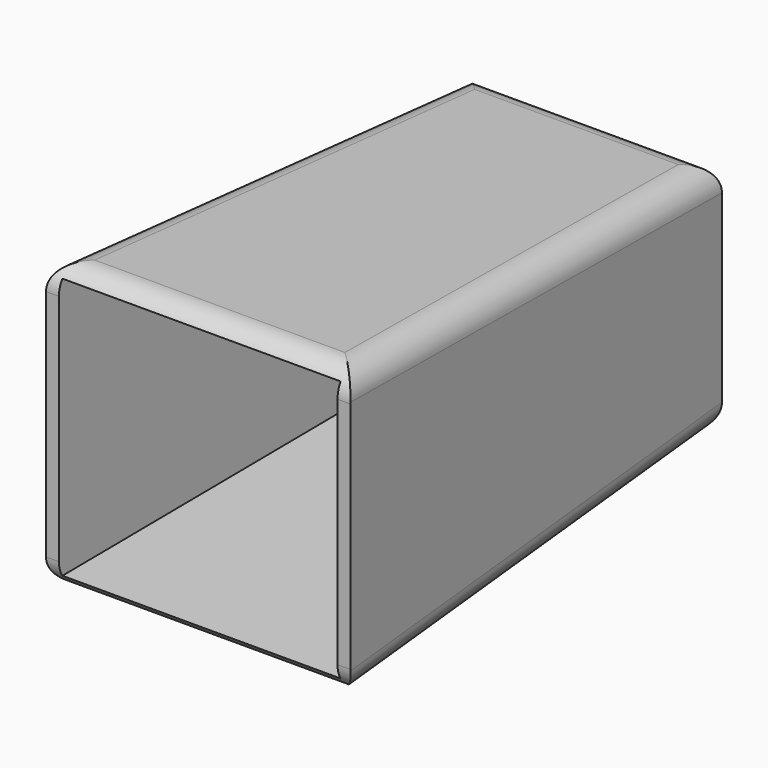
from build123d import *

# Parameters (mm, degrees)
F0_W        = 50
F0_H        = 46.7033070608
F1_DEPTH    = 98.552
F1_TAPER    = -3
F2_T        = -2.54
F3_T1_DEPTH = 74.1036999946
F3_T3_DEPTH = 124.1528328785
F3_T5_DEPTH = 87.0957981099
F3_T7_DEPTH = 124.1528328785
F4_T1_DEPTH = 74.1036999946
F4_T3_DEPTH = 124.1528328785
F4_T5_DEPTH = 87.0957981099
F4_T7_DEPTH = 124.1528328785


# Not quite as in the source:
# - a fillet or chamfer that OpenCascade refuses, or shapes differently, is made with other operations: its cross-section is extruded or revolved along the edge and cut away or added


with BuildPart() as f1:
    # F0 (on Front) → F1 (new body)
    with BuildSketch(Plane.XZ):
        Rectangle(F0_W, F0_H)
    extrude(amount=F1_DEPTH, taper=F1_TAPER)

    # F2
    f2_openings = [f1.faces().sort_by_distance(p)[0] for p in [
        (0, -98.552, 0),
    ]]
    offset(amount=F2_T, openings=f2_openings)

    # F3: fillet of radius 5.08 on 4 edges, made by hand

    # F3_s2 → F3_t1 (cut)
    with BuildSketch(Plane.YZ.offset(-37.0518499973)):
        with BuildLine():
            ThreePointArc((-4.8141333423, 23.6039515681), (-1.3950981953, 22.027754776), (0, 18.5309135315))
            Line((0, 18.5309135315), (0, 23.3516535304))
            Line((0, 23.3516535304), (-4.8141333423, 23.6039515681))
        make_face()
    extrude(amount=F3_T1_DEPTH, mode=Mode.SUBTRACT)

    # F3_s4 → F3_t3 (cut)
    with BuildSketch(Plane(origin=(0.5298667006, 10.1104589396, -0.5298667006), x_dir=(0.9986295348, -0.0523359562, 0), z_dir=(-0.0522644277, -0.9972646886, 0.0522644277))):
        with BuildLine():
            ThreePointArc((-24.9657383689, 18.1852510398), (-23.4827569315, 21.7724306367), (-19.8996527546, 23.2652319837))
            Line((-19.8996527546, 23.2652319837), (-24.9657383689, 23.2513556581))
            Line((-24.9657383689, 23.2513556581), (-24.9657383689, 18.1852510398))
        make_face()
    extrude(amount=F3_T3_DEPTH, mode=Mode.SUBTRACT)

    # F3_s6 → F3_t5 (cut)
    with BuildSketch(Plane.YZ.offset(-43.547899055)):
        with BuildLine():
            ThreePointArc((-93.2061333423, 28.2363799944), (-96.9688412445, 26.8482437626), (-98.552, 23.1633419579))
            Line((-98.552, 23.1633419579), (-98.552, 28.5165449943))
            Line((-98.552, 28.5165449943), (-93.2061333423, 28.2363799944))
        make_face()
    extrude(amount=F3_T5_DEPTH, mode=Mode.SUBTRACT)

    # F3_s8 → F3_t7 (cut)
    with BuildSketch(Plane(origin=(-0.5298667006, 10.1104589396, -0.5298667006), x_dir=(0.9986295348, 0.0523359562, 0), z_dir=(0.0522644277, -0.9972646886, 0.0522644277))):
        with BuildLine():
            ThreePointArc((24.9657383689, 18.1852510398), (23.4827569315, 21.7724306367), (19.8996527546, 23.2652319837))
            Line((19.8996527546, 23.2652319837), (24.9657383689, 23.2513556581))
            Line((24.9657383689, 23.2513556581), (24.9657383689, 18.1852510398))
        make_face()
    extrude(amount=F3_T7_DEPTH, mode=Mode.SUBTRACT)

    # F4: fillet of radius 5.08 on 4 edges, made by hand

    # F4_s2 → F4_t1 (cut)
    with BuildSketch(Plane.YZ.offset(-37.0518499973)):
        with BuildLine():
            ThreePointArc((-4.8141333423, -23.6039515681), (-1.3950981953, -22.027754776), (0, -18.5309135315))
            Line((0, -18.5309135315), (0, -23.3516535304))
            Line((0, -23.3516535304), (-4.8141333423, -23.6039515681))
        make_face()
    extrude(amount=F4_T1_DEPTH, mode=Mode.SUBTRACT)

    # F4_s4 → F4_t3 (cut)
    with BuildSketch(Plane(origin=(-0.5298667006, 10.1104589396, 0.5298667006), x_dir=(0.9986295348, 0.0523359562, 0), z_dir=(0.0522644277, -0.9972646886, -0.0522644277))):
        with BuildLine():
            ThreePointArc((19.8996527546, -23.2652319837), (23.4827569315, -21.7724306367), (24.9657383689, -18.1852510398))
            Line((24.9657383689, -18.1852510398), (24.9657383689, -23.2513556581))
            Line((24.9657383689, -23.2513556581), (19.8996527546, -23.2652319837))
        make_face()
    extrude(amount=F4_T3_DEPTH, mode=Mode.SUBTRACT)

    # F4_s6 → F4_t5 (cut)
    with BuildSketch(Plane.YZ.offset(-43.547899055)):
        with BuildLine():
            ThreePointArc((-98.552, -23.1633419579), (-96.9688412445, -26.8482437626), (-93.2061333423, -28.2363799944))
            Line((-93.2061333423, -28.2363799944), (-98.552, -28.5165449943))
            Line((-98.552, -28.5165449943), (-98.552, -23.1633419579))
        make_face()
    extrude(amount=F4_T5_DEPTH, mode=Mode.SUBTRACT)

    # F4_s8 → F4_t7 (cut)
    with BuildSketch(Plane(origin=(0.5298667006, 10.1104589396, 0.5298667006), x_dir=(0.9986295348, -0.0523359562, 0), z_dir=(-0.0522644277, -0.9972646886, -0.0522644277))):
        with BuildLine():
            ThreePointArc((-24.9657383689, -18.1852510398), (-23.4827569315, -21.7724306367), (-19.8996527546, -23.2652319837))
            Line((-19.8996527546, -23.2652319837), (-24.9657383689, -23.2513556581))
            Line((-24.9657383689, -23.2513556581), (-24.9657383689, -18.1852510398))
        make_face()
    extrude(amount=F4_T7_DEPTH, mode=Mode.SUBTRACT)


solid = f1.part
